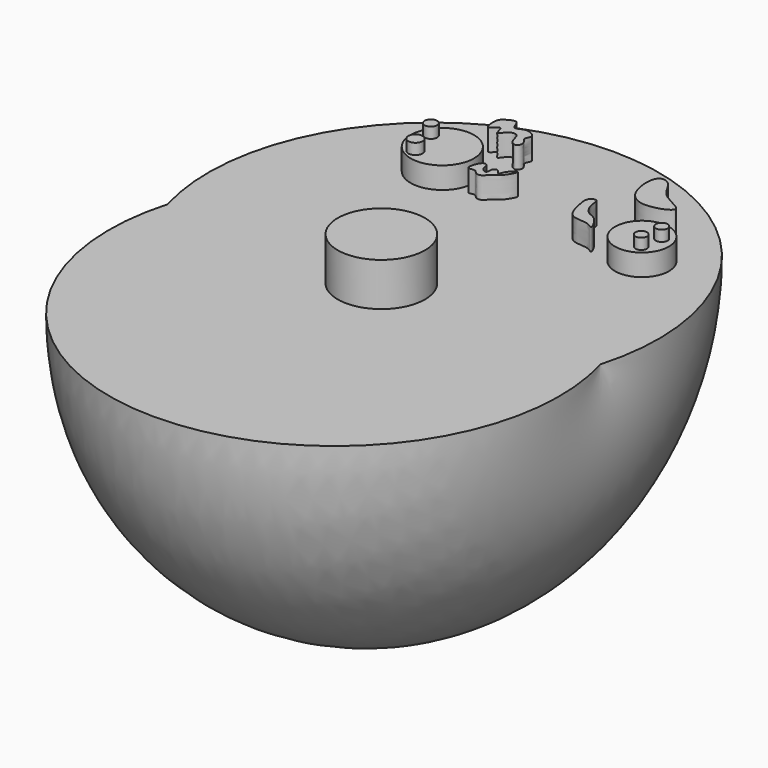
from build123d import *

# Parameters (mm, degrees)
F1_ANGLE  = 180
F2_R      = 4.0305965855
F3_DEPTH  = 4
F7_R      = 2.4890400521
F8_DEPTH  = 2
F9_R      = 2.92739538
F10_DEPTH = 2
F12_R     = 0.5323906091
F13_DEPTH = 1
F14_R     = 0.5428831827
F15_DEPTH = 1
F17_R     = 0.660648137
F18_DEPTH = 1
F19_R     = 0.572209203
F20_DEPTH = 1
F22_DEPTH = 2
F24_DEPTH = 2
F26_DEPTH = 2
F28_DEPTH = 2


# Not quite as in the source:
# - the program builds the solid bodies; features that only make, move or delete a surface that nothing else refers to are left out


with BuildPart() as f1:
    # F0 (on Top) → F1 (revolve)
    with BuildSketch(Plane.XY):
        with BuildLine():
            Line((-40, 0), (0, 0))
            ThreePointArc((0, 0), (-20, 26.5239931319), (-40, 0))
        make_face()
    revolve(axis=Axis((-20, 0, 0), (-1, 0, 0)), revolution_arc=F1_ANGLE)

    # F2 (on Top) → F3 (join)
    with BuildSketch(Plane.XY):
        with Locations((-20.244076848, 0)):
            Circle(F2_R)
    extrude(amount=F3_DEPTH)

    # F7 (on face) → F8 (join)
    with BuildSketch(Plane.XY):
        with Locations((-7.7222660184, 14.4360847771)):
            Circle(F7_R)
    extrude(amount=F8_DEPTH)

    # F9 (on face) → F10 (join)
    with BuildSketch(Plane.XY):
        with Locations((-27.7437642217, 16.4119936526)):
            Circle(F9_R)
    extrude(amount=F10_DEPTH)

    # F12 (on face) → F13 (join)
    with BuildSketch(Plane.XY.offset(2)):
        with Locations((-6.7914389074, 13.187520206)):
            Circle(F12_R)
    extrude(amount=F13_DEPTH)

    # F14 (on face) → F15 (join)
    with BuildSketch(Plane.XY.offset(2)):
        with Locations((-6.422534585, 15.091329813)):
            Circle(F14_R)
    extrude(amount=F15_DEPTH)

    # F17 (on face) → F18 (join)
    with BuildSketch(Plane.XY.offset(2)):
        with Locations((-28.8453288376, 14.6901383996)):
            Circle(F17_R)
    extrude(amount=F18_DEPTH)

    # F19 (on face) → F20 (join)
    with BuildSketch(Plane.XY.offset(2)):
        with Locations((-29.4963382185, 17.2892063856)):
            Circle(F19_R)
    extrude(amount=F20_DEPTH)

    # F21 (on face) → F22 (join)
    with BuildSketch(Plane.XY):
        with BuildLine():
            add(Edge.make_bspline(
                [(-8.5160620511, 19.3127393723), (-8.521972931, 19.6839333445), (-10.7305748769, 20.2704778577), (-11.1816446669, 22.2750778583), (-12.9097861424, 22.6512643434), (-12.7707594725, 19.3129856124), (-10.8028333219, 18.0206741983), (-8.5100583053, 18.9357135717), (-8.5160620511, 19.3127393723)],
                knots=[0, 0, 0, 0, 0.1722414989, 0.3410756935, 0.4579261422, 0.6476969394, 0.825052415, 1, 1, 1, 1], degree=3))
        make_face()
    extrude(amount=F22_DEPTH)

    # F23 (on face) → F24 (join)
    with BuildSketch(Plane.XY):
        with BuildLine():
            add(Edge.make_bspline(
                [(-11.5098860115, 13.2981240749), (-11.457220893, 13.3937996973), (-12.1204864542, 14.7306910435), (-13.1118095158, 14.7779928006), (-13.7607902099, 15.9868173482), (-13.6541299737, 16.9766064821), (-14.5890741737, 16.7131041232), (-14.4044989561, 15.4604322823), (-13.8847921779, 13.4671527284), (-12.1299745641, 13.808764838), (-11.5457660553, 13.2329415476), (-11.5098860115, 13.2981240749)],
                knots=[0, 0, 0, 0, 0.1229696245, 0.2306521994, 0.3507800699, 0.4446437385, 0.522990954, 0.6383534919, 0.7819443294, 0.9162224325, 1, 1, 1, 1], degree=3))
        make_face()
    extrude(amount=F24_DEPTH)

    # F25 (on face) → F26 (join)
    with BuildSketch(Plane.XY):
        with BuildLine():
            add(Edge.make_bspline(
                [(-27.0097907633, 20.8374261856), (-27.2425727265, 20.8319652886), (-27.4031250895, 22.1733922891), (-26.8329748697, 22.5675757298), (-25.7995869833, 23.0916938033), (-25.7024529374, 21.6580021561), (-24.804928822, 22.2635565151), (-24.2649902936, 22.1929586914), (-23.4683819898, 21.7214432552), (-24.1302189882, 21.0623235273), (-23.3146935561, 20.5271971589), (-23.7432502692, 19.6969266917), (-24.5258521864, 20.2940513308), (-24.4662124217, 21.3036490589), (-25.5311996305, 21.3355170611), (-26.0520117333, 20.0392582092), (-26.2152630753, 21.9090074999), (-26.813783683, 20.8420243704), (-27.0097907633, 20.8374261856)],
                knots=[0, 0, 0, 0, 0.0771030843, 0.1400826747, 0.2042110914, 0.2710483491, 0.3319249501, 0.387198642, 0.4464269542, 0.5018605974, 0.563334419, 0.6177911928, 0.6778378112, 0.7441908676, 0.8070383996, 0.8697787648, 0.9350776572, 1, 1, 1, 1], degree=3))
        make_face()
    extrude(amount=F26_DEPTH)

    # F27 (on face) → F28 (join)
    with BuildSketch(Plane.XY):
        with BuildLine():
            add(Edge.make_bspline(
                [(-24.2265574634, 15.0205790997), (-24.1248145615, 14.8875807453), (-23.5647992126, 15.1811169827), (-23.2781166392, 14.5787051468), (-22.6390340236, 14.6349514416), (-22.3040150935, 15.2195858598), (-21.6699712546, 15.5437359225), (-21.2757359012, 16.0472006168), (-20.7833567862, 17.0586009621), (-21.8285044828, 16.2313624992), (-21.9211040318, 15.3975196089), (-22.3291080033, 16.2071935321), (-22.8193786359, 15.9176745538), (-22.6537006109, 15.0747834744), (-23.4586142076, 15.5827339886), (-23.314763112, 16.1318993459), (-23.9815444448, 16.5043044772), (-24.3771186928, 15.2173927876), (-24.2265574634, 15.0205790997)],
                knots=[0, 0, 0, 0, 0.0606105338, 0.1191364942, 0.1759327084, 0.2398484718, 0.3054555849, 0.3741341104, 0.437667682, 0.5128748319, 0.5727520461, 0.6313351165, 0.6804198879, 0.7405122341, 0.8005084259, 0.8583877769, 0.9103072911, 1, 1, 1, 1], degree=3))
        make_face()
    extrude(amount=F28_DEPTH)


solid = f1.part
